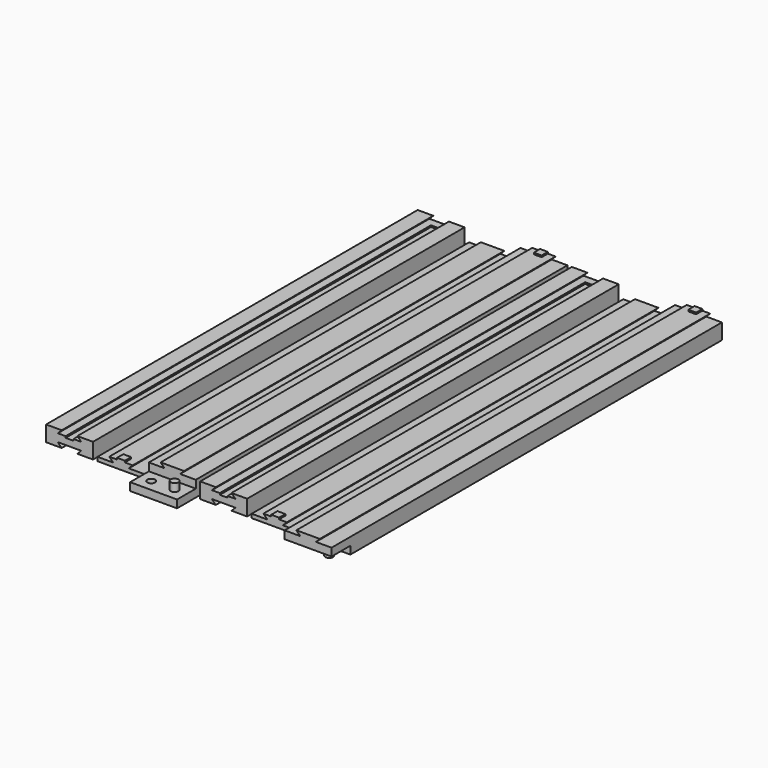
from build123d import *

# Parameters (mm, degrees)
F0_W        = 30
F0_H        = 10
F1_DEPTH    = 297
F3_DEPTH    = 297
F5_DEPTH    = 297
F7_DEPTH    = 297
F8_W        = 5
F8_H        = 5
F9_DEPTH    = 1
F10_W       = 5
F10_H       = 292
F11_DEPTH   = 1
F13_DEPTH   = 297
F15_W       = 5
F15_H       = 1
F16_DEPTH   = 292
F17_W       = 30
F17_H       = 297
F18_DEPTH   = 7.5
F19_W       = 5
F19_H       = 292
F20_DEPTH   = 1
F21_W       = 15
F21_H       = 5
F22_DEPTH   = 15
F23_R       = 2.5
F24_DEPTH   = 5.001
F25_DEPTH   = 5
F28_FACE1_R = 2.5
F29_W       = 30
F29_H       = 15
F29_R       = 2.5
F30_DEPTH   = 25.4
F32_DEPTH   = 15
F33_R       = 2.5
F34_DEPTH   = 5
F35_DEPTH   = 5
F36_ANGLE   = 270


# Not quite as in the source:
# - a feature names something its author has since deleted; it is built from what else it names


with BuildPart() as f1:
    # F0 (on Top) → F1 (new body)
    with BuildSketch(Plane.XY):
        Rectangle(F0_W, F0_H)
    extrude(amount=F1_DEPTH)

    # F2 (on face) → F3 (cut)
    with BuildSketch(Plane.XY.offset(297)):
        Polygon((7.5, 2.5), (5, 5), (-5, 5), (-7.5, 2.5), align=None)
        Polygon((-5, -5), (5, -5), (7.5, -2.5), (-7.5, -2.5), align=None)
    extrude(amount=-F3_DEPTH, mode=Mode.SUBTRACT)

    # F10 (on face) → F11 (cut)
    with BuildSketch(Plane(origin=(0, 2.5, 0), x_dir=(-1, 0, 0), z_dir=(0, 1, 0))):
        with Locations((0, 151)):
            Rectangle(F10_W, F10_H)
    extrude(amount=-F11_DEPTH, mode=Mode.SUBTRACT)

    # F19 (on face) → F20 (cut)
    with BuildSketch(Plane.XZ.offset(2.5)):
        with Locations((0, 146)):
            Rectangle(F19_W, F19_H)
    extrude(amount=-F20_DEPTH, mode=Mode.SUBTRACT)


with BuildPart() as f5:
    # F4 (on Top) → F5 (new body)
    with BuildSketch(Plane.XY):
        Polygon((40.3872628876, 5), (25.3872628876, 5), (27.8872628876, 2.5), (37.8872628876, 2.5), align=None)
        Polygon((27.8872628876, 2.5), (17.8872628876, 2.5), (17.8872628876, 0), (47.8872628876, 0), (47.8872628876, 2.5), (37.8872628876, 2.5), align=None)
        Polygon((25.3872628876, 5), (17.8872628876, 5), (17.8872628876, 2.5), (27.8872628876, 2.5), align=None)
        Polygon((47.8872628876, 5), (40.3872628876, 5), (37.8872628876, 2.5), (47.8872628876, 2.5), align=None)
    extrude(amount=F5_DEPTH)

    # F6 (on face) → F7 (cut)
    with BuildSketch(Plane.XY.offset(297)):
        Polygon((17.8872628876, 2.5), (27.8872628876, 2.5), (25.3872628876, 5), (17.8872628876, 5), align=None)
        Polygon((40.3872628876, 5), (37.8872628876, 2.5), (47.8872628876, 2.5), (47.8872628876, 5), align=None)
    extrude(amount=-F7_DEPTH, mode=Mode.SUBTRACT)

    # F8 (on face) → F9 (join)
    with BuildSketch(Plane(origin=(0, 5, 0), x_dir=(-1, 0, 0), z_dir=(0, 1, 0))):
        with Locations((-32.8872628876, 294.5)):
            Rectangle(F8_W, F8_H)
    extrude(amount=F9_DEPTH)


with BuildPart() as f13:
    # F12 (on face) → F13 (new body)
    with BuildSketch(Plane.XY.offset(297)):
        Polygon((50.7294392586, 2.5), (50.7294392586, 0), (80.7294392586, 0), (80.7294392586, 2.5), (70.7294392586, 2.5), (73.2294392586, 5), (68.2294392586, 5), (68.2294392586, 6), (63.2294392586, 6), (63.2294392586, 5), (58.2294392586, 5), (60.7294392586, 2.5), align=None)
    extrude(amount=F13_DEPTH)


with BuildPart() as f13_1:
    # F14: moved
    add(f13.part.moved(Location((0, 0, -297))))

    # F15 (on face) → F16 (cut)
    with BuildSketch(Plane.XY.offset(297)):
        with Locations((65.7294392586, 5.5)):
            Rectangle(F15_W, F15_H)
    extrude(amount=-F16_DEPTH, mode=Mode.SUBTRACT)

    # F17 (on face) → F18 (join)
    with BuildSketch(Plane.XZ):
        with Locations((65.7294392586, 148.5)):
            Rectangle(F17_W, F17_H)
    extrude(amount=F18_DEPTH)

    # F21 (on face) → F22 (join)
    with BuildSketch(Plane.XY.offset(297)):
        with Locations((58.2294392586, -5)):
            Rectangle(F21_W, F21_H)
        with Locations((73.2294392586, -5)):
            Rectangle(F21_W, F21_H)
    extrude(amount=F22_DEPTH)

    # F23 (on face) → F24 (cut, through all)
    with BuildSketch(Plane(origin=(0, -2.5, 0), x_dir=(-1, 0, 0), z_dir=(0, 1, 0))):
        with Locations((-58.2294392586, 304.5)):
            Circle(F23_R)
    extrude(amount=-F24_DEPTH, mode=Mode.SUBTRACT)

    # F23 (on face) → F25 (join)
    with BuildSketch(Plane(origin=(0, -2.5, 0), x_dir=(-1, 0, 0), z_dir=(0, 1, 0))):
        with Locations((-73.2294392586, 304.5)):
            Circle(F23_R)
    extrude(amount=F25_DEPTH)


with BuildPart() as f26_1:
    # F26: copy of F1
    add(f1.part.moved(Location((188.468, 0, 0))))


with BuildPart() as f26_2:
    # F26: copy of F5
    add(f5.part.moved(Location((188.468, 0, 0))))


with BuildPart() as f26_3:
    # F26: copy of F13
    add(f13_1.part.moved(Location((188.468, 0, 0))))


with BuildPart() as f28_1:
    # F28: copy of F13
    add(f13_1.part.moved(Location((207.264, 0, 0))))

    # F28_face1 (on face) + F29 (on face) → F30 (cut)
    with BuildSketch(Plane(origin=(280.4934392586, 2.5, 304.5), x_dir=(-1, 0, 0), z_dir=(0, 1, 0))):
        Circle(F28_FACE1_R)
    with BuildSketch(Plane(origin=(0, -2.5, 0), x_dir=(-1, 0, 0), z_dir=(0, 1, 0))):
        with Locations((-272.9934392586, 304.5)):
            Rectangle(F29_W, F29_H)
        with Locations((-280.4934392586, 304.5)):
            Circle(F29_R, mode=Mode.SUBTRACT)
        with Locations((-265.4934392586, 304.5)):
            Circle(F29_R, mode=Mode.SUBTRACT)
    extrude(amount=-F30_DEPTH, mode=Mode.SUBTRACT)

    # F31 (on face) → F32 (join)
    with BuildSketch(Plane.XY.offset(297)):
        Polygon((257.9934392586, 2.5), (257.9934392586, -2.5), (287.9934392586, -2.5), (287.9934392586, 2.5), (277.9934392586, 2.5), (280.4934392586, 5), (265.4934392586, 5), (267.9934392586, 2.5), align=None)
    extrude(amount=F32_DEPTH)

    # F33 (on face) → F34 (join)
    with BuildSketch(Plane.XZ.offset(2.5)):
        with Locations((280.4934392586, 304.5)):
            Circle(F33_R)
    extrude(amount=F34_DEPTH)

    # F33 (on face) → F35 (cut)
    with BuildSketch(Plane.XZ.offset(2.5)):
        with Locations((265.4934392586, 304.5)):
            Circle(F33_R)
    extrude(amount=-F35_DEPTH, mode=Mode.SUBTRACT)


with BuildPart() as f1_1:
    # F36: moved
    add(f1.part.rotate(Axis((10, -5, 0), (-1, 0, 0)), F36_ANGLE))


with BuildPart() as f5_1:
    # F36: moved
    add(f5.part.rotate(Axis((10, -5, 0), (-1, 0, 0)), F36_ANGLE))


with BuildPart() as f13_2:
    # F36: moved
    add(f13_1.part.rotate(Axis((10, -5, 0), (-1, 0, 0)), F36_ANGLE))


with BuildPart() as f26_1_1:
    # F36: moved
    add(f26_1.part.rotate(Axis((10, -5, 0), (-1, 0, 0)), F36_ANGLE))


with BuildPart() as f26_2_1:
    # F36: moved
    add(f26_2.part.rotate(Axis((10, -5, 0), (-1, 0, 0)), F36_ANGLE))


with BuildPart() as f28_1_1:
    # F36: moved
    add(f28_1.part.rotate(Axis((10, -5, 0), (-1, 0, 0)), F36_ANGLE))


with BuildPart() as f28_1_2:
    # F37: moved
    add(f28_1_1.part.moved(Location((-18.542, 0, 0))))


with BuildPart() as f26_1_2:
    # F38: moved
    add(f26_1_1.part.moved(Location((-89.916, 0, 0))))


with BuildPart() as f26_2_2:
    # F38: moved
    add(f26_2_1.part.moved(Location((-89.916, 0, 0))))


with BuildPart() as f28_1_3:
    # F38: moved
    add(f28_1_2.part.moved(Location((-89.916, 0, 0))))


with BuildPart() as f5_2:
    # F39: moved
    add(f5_1.part.moved(Location((0, 0, -5))))


with BuildPart() as f26_2_3:
    # F39: moved
    add(f26_2_2.part.moved(Location((0, 0, -5))))


with BuildPart() as f13_3:
    # F40: moved
    add(f13_2.part.moved(Location((0, 0, 2.5))))


with BuildPart() as f28_1_4:
    # F40: moved
    add(f28_1_3.part.moved(Location((0, 0, 2.5))))


with BuildPart() as f1_2:
    # F41: moved
    add(f1_1.part.moved(Location((-78.994, 162.814, 0))))


with BuildPart() as f5_3:
    # F41: moved
    add(f5_2.part.moved(Location((-78.994, 162.814, 0))))


with BuildPart() as f13_4:
    # F41: moved
    add(f13_3.part.moved(Location((-78.994, 162.814, 0))))


with BuildPart() as f26_1_3:
    # F41: moved
    add(f26_1_2.part.moved(Location((-78.994, 162.814, 0))))


with BuildPart() as f26_2_4:
    # F41: moved
    add(f26_2_3.part.moved(Location((-78.994, 162.814, 0))))


with BuildPart() as f28_1_5:
    # F41: moved
    add(f28_1_4.part.moved(Location((-78.994, 162.814, 0))))


solid = Compound([f1_2.part, f5_3.part, f13_4.part, f26_1_3.part, f26_2_4.part, f28_1_5.part])
